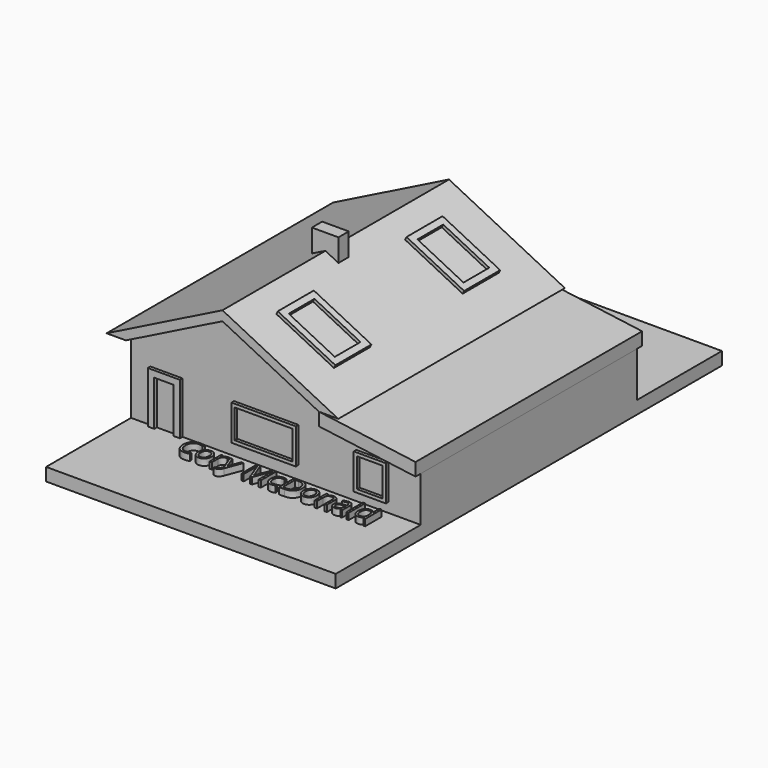
from build123d import *

# Parameters (mm, degrees)
F1_DEPTH      = 6705.6
F0_W          = 3048
F0_H          = 1676.4
F0_W_2        = 1524
F2_DEPTH      = 6400.8
F0_W_3        = 4572
F0_H_2        = 609.6
F3_DEPTH      = 11430
F0_W_4        = 1219.2
F0_H_3        = 1371.6
F4_DEPTH      = 6400.8
F0_W_5        = 2743.2
F5_DEPTH      = 6553.2
F6_DEPTH      = 6553.2
F0_W_6        = 914.4
F0_H_4        = 2133.6
F7_DEPTH      = 6400.8
F8_W          = 1524
F8_H          = 1676.4
F8_W_2        = 914.4
F8_H_2        = 1066.8
F9_DEPTH      = 3.048
F10_DEPTH     = 6400.8
F11_DEPTH     = 6553.2
F12_DEPTH     = 152.4
F13_DEPTH     = 30.48
F14_W         = 3048
F14_H         = 2133.6
F14_W_2       = 2438.4
F14_H_2       = 1524
F15_DEPTH     = 152.4
F16_W         = 2991.4143345833
F16_H         = 2513.076
F16_W_2       = 2686.6143345833
F16_H_2       = 2208.276
F16_W_3       = 2991.3072
F16_H_3       = 2513.1688378334
F16_W_4       = 2686.5072
F16_H_4       = 2208.3688378334
F17_DEPTH     = 152.4
F18_DEPTH     = 609.6
F19_TEXT_SIZE = 1281.8223633775
F20_DEPTH     = 304.8


# Not quite as in the source:
# - Text() gives the source's letters only with a copy of the font that has no kerning and outlines rounded to 1/6400 em; it was checked with that copy


with BuildPart() as f1:
    # F0 (on Front) → F1 (new body, symmetric)
    with BuildSketch(Plane.XZ):
        Polygon((0, 2286), (4572, 0), (5486.4, 0), (616.0258992004, 2435.1870503998), (0, 2743.2), align=None)
        Polygon((-5486.4, 0), (-4572, 0), (0, 2286), (0, 2743.2), (-640.9901380539, 2422.7049309731), align=None)
    extrude(amount=F1_DEPTH, both=True)

    # F14 (on face) → F15 (join)
    with BuildSketch(Plane(origin=(1097.28, 0, 2194.56), x_dir=(0.894427191, 0, -0.4472135955), z_dir=(0.4472135955, 0, 0.894427191))):
        with Locations((1516.4036648245, 3810)):
            Rectangle(F14_W, F14_H)
        with Locations((1516.4036648245, 3810)):
            Rectangle(F14_W_2, F14_H_2, mode=Mode.SUBTRACT)
        with Locations((1516.4036648245, -3810)):
            Rectangle(F14_W, F14_H)
        with Locations((1516.4036648245, -3810)):
            Rectangle(F14_W_2, F14_H_2, mode=Mode.SUBTRACT)
    extrude(amount=F15_DEPTH)

    # F0 (on Front) → F18 (join)
    with BuildSketch(Plane.XZ):
        Polygon((-640.9901380539, 2422.7049309731), (0, 2743.2), (616.0258992004, 2435.1870503998), (616.0258992004, 3505.3545309731), (-640.9901380539, 3505.3545309731), align=None)
    extrude(amount=F18_DEPTH)


with BuildPart() as f1b:
    # F0 (on Front) → F1, piece 2 (new body, symmetric)
    with BuildSketch(Plane.XZ):
        Polygon((9144, -609.6), (4572, 0), (4572, -609.6), (9144, -1219.2), align=None)
    extrude(amount=F1_DEPTH, both=True)


with BuildPart() as f2:
    # F0 (on Front) → F2 (new body, symmetric)
    with BuildSketch(Plane.XZ):
        Polygon((-4572, 0), (0, 0), (0, 2286), align=None)
        Polygon((0, 2286), (0, 0), (4572, 0), align=None)
        Polygon((4572, 0), (0, 0), (-4572, 0), (-4572, -3352.8), (-3657.6, -3352.8), (-3657.6, -914.4), (-2133.6, -914.4), (-2133.6, -3352.8), (4572, -3352.8), (4572, -609.6), align=None)
        with Locations((1828.8, -1905)):
            Rectangle(F0_W, F0_H, mode=Mode.SUBTRACT)
        Polygon((9144, -1219.2), (4572, -609.6), (4572, -3352.8), (9144, -3352.8), align=None)
        with Locations((6858, -2057.4)):
            Rectangle(F0_W_2, F0_H, mode=Mode.SUBTRACT)
    extrude(amount=F2_DEPTH, both=True)

    # F0 (on Front) → F3 (join, symmetric)
    with BuildSketch(Plane.XZ):
        with Locations((6858, -3657.6)):
            Rectangle(F0_W_3, F0_H_2)
        Polygon((-3657.6, -3352.8), (-4572, -3352.8), (-4572, -3962.4), (4572, -3962.4), (4572, -3352.8), (-2133.6, -3352.8), (-2438.4, -3352.8), (-3352.8, -3352.8), align=None)
    extrude(amount=F3_DEPTH, both=True)

    # F0 (on Front) → F6 (join, symmetric)
    with BuildSketch(Plane.XZ):
        Polygon((-3657.6, -914.4), (-3657.6, -3352.8), (-3352.8, -3352.8), (-3352.8, -1219.2), (-2438.4, -1219.2), (-2438.4, -3352.8), (-2133.6, -3352.8), (-2133.6, -914.4), align=None)
    extrude(amount=F6_DEPTH, both=True)

    # F0 (on Front) → F7 (join, symmetric)
    with BuildSketch(Plane.XZ):
        with Locations((-2895.6, -2286)):
            Rectangle(F0_W_6, F0_H_4)
    extrude(amount=F7_DEPTH, both=True)

    # F16 (on face) → F17 (join)
    with BuildSketch(Plane(origin=(-4572, 0, 0), x_dir=(0, -1, 0), z_dir=(-1, 0, 0))):
        with Locations((3533.4928327084, -2018.538)):
            Rectangle(F16_W, F16_H)
        with Locations((3533.4928327084, -2018.538)):
            Rectangle(F16_W_2, F16_H_2, mode=Mode.SUBTRACT)
        with Locations((-3533.5464, -2018.5844189167)):
            Rectangle(F16_W_3, F16_H_3)
        with Locations((-3533.5464, -2018.5844189167)):
            Rectangle(F16_W_4, F16_H_4, mode=Mode.SUBTRACT)
    extrude(amount=F17_DEPTH)

    # F19 (on face) → F20 (join)
    with BuildSketch(Plane.XY.offset(-3352.8)):
        with Locations((-1447.4801192874, -7772.4)):
            Text('Cory McDonald', F19_TEXT_SIZE, font='Open Sans', text_align=(TextAlign.LEFT, TextAlign.BOTTOM))
    extrude(amount=F20_DEPTH)


with BuildPart() as f4:
    # F0 (on Front) → F4 (new body)
    with BuildSketch(Plane.XZ):
        with Locations((6858, -2057.4)):
            Rectangle(F0_W_4, F0_H_3)
    extrude(amount=F4_DEPTH)


with BuildPart() as f4b:
    # F0 (on Front) → F4, piece 2 (new body)
    with BuildSketch(Plane.XZ):
        with Locations((1828.8, -1905)):
            Rectangle(F0_W_5, F0_H_3)
    extrude(amount=F4_DEPTH)

    # F10 (add): a face of the model
    f10_faces = [f4b.faces().sort_by_distance(p)[0] for p in [
        (1828.8, 0, -1905),
    ]]
    extrude(f10_faces, amount=F10_DEPTH)


with BuildPart() as f5:
    # F0 (on Front) → F5 (new body)
    with BuildSketch(Plane.XZ):
        with Locations((1828.8, -1905)):
            Rectangle(F0_W, F0_H)
        with Locations((1828.8, -1905)):
            Rectangle(F0_W_5, F0_H_3, mode=Mode.SUBTRACT)
    extrude(amount=F5_DEPTH)


with BuildPart() as f5b:
    # F0 (on Front) → F5, piece 2 (new body)
    with BuildSketch(Plane.XZ):
        with Locations((6858, -2057.4)):
            Rectangle(F0_W_2, F0_H)
        with Locations((6858, -2057.4)):
            Rectangle(F0_W_4, F0_H_3, mode=Mode.SUBTRACT)
    extrude(amount=F5_DEPTH)


with BuildPart() as f9:
    # F8 (on face) → F9 (new body)
    with BuildSketch(Plane(origin=(0, 6400.8, 0), x_dir=(-1, 0, 0), z_dir=(0, 1, 0))):
        with Locations((-6858, -2057.4)):
            Rectangle(F8_W, F8_H)
        with Locations((-6858, -2057.4)):
            Rectangle(F8_W_2, F8_H_2, mode=Mode.SUBTRACT)
    extrude(amount=F9_DEPTH)

    # F8 (on face) → F12 (join)
    with BuildSketch(Plane(origin=(0, 6400.8, 0), x_dir=(-1, 0, 0), z_dir=(0, 1, 0))):
        with Locations((-6858, -2057.4)):
            Rectangle(F8_W, F8_H)
        with Locations((-6858, -2057.4)):
            Rectangle(F8_W_2, F8_H_2, mode=Mode.SUBTRACT)
    extrude(amount=F12_DEPTH)

    # F8 (on face) → F13 (join)
    with BuildSketch(Plane(origin=(0, 6400.8, 0), x_dir=(-1, 0, 0), z_dir=(0, 1, 0))):
        with Locations((-6858, -2057.4)):
            Rectangle(F8_W_2, F8_H_2)
    extrude(amount=F13_DEPTH)


with BuildPart() as f11:
    # F11 (new): a face of the model
    f11_faces = [f5.part.faces().sort_by_distance(p)[0] for p in [
        (1828.8, 0, -1101.5859468176),
    ]]
    extrude(f11_faces, amount=F11_DEPTH)


solid = Compound([f1.part, f1b.part, f2.part, f4.part, f4b.part, f5.part, f5b.part, f9.part, f11.part])
